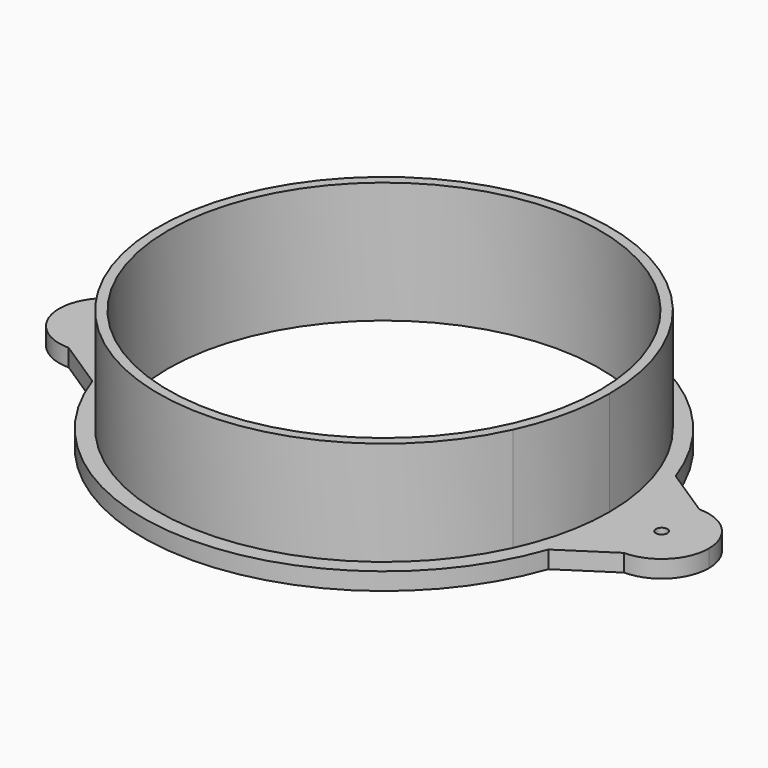
from build123d import *

# Parameters (mm, degrees)
F1_DEPTH = 5
F0_R     = 1.6686337588
F2_DEPTH = 5
F3_DEPTH = 35


with BuildPart() as f1:
    # F0 (on Top) → F1 (new body)
    with BuildSketch(Plane.XY):
        with BuildLine():
            ThreePointArc((58.9908692784, -27.2961048829), (63.4799436952, -13.9748613035), (65, 0))
            ThreePointArc((65, 0), (63.4799436952, 13.9748613035), (58.9908692784, 27.2961048829))
            ThreePointArc((58.9908692784, 27.2961048829), (35.0053794624, 54.7688178501), (0, 65))
            ThreePointArc((0, 65), (-35.0053794624, 54.7688178501), (-58.9908692784, 27.2961048829))
            ThreePointArc((-58.9908692784, 27.2961048829), (-63.4799436952, 13.9748613035), (-65, 0))
            ThreePointArc((-65, 0), (-63.4799436952, -13.9748613035), (-58.9908692784, -27.2961048829))
            ThreePointArc((-58.9908692784, -27.2961048829), (0, -65), (58.9908692784, -27.2961048829))
        make_face()
        with BuildLine():
            ThreePointArc((-62.231150434, 0), (-44.0040684729, 44.0040684729), (0, 62.231150434))
            ThreePointArc((0, 62.231150434), (44.0040684729, 44.0040684729), (62.231150434, 0))
            ThreePointArc((62.231150434, 0), (0, -62.231150434), (-62.231150434, 0))
        make_face(mode=Mode.SUBTRACT)
        with BuildLine():
            ThreePointArc((58.9908692784, 27.2961048829), (63.4799436952, 13.9748613035), (65, 0))
            Line((65, 0), (66.4206601738, 0))
            ThreePointArc((66.4206601738, 0), (67.1091179562, 4.268914411), (69.1046831796, 8.1049701726))
            ThreePointArc((69.1046831796, 8.1049701726), (67.8057771791, 15.6052670592), (65.6953330705, 22.9187912336))
            Line((65.6953330705, 22.9187912336), (58.9908692784, 27.2961048829))
        make_face()
        with BuildLine():
            Line((66.4206601738, 0), (65, 0))
            ThreePointArc((65, 0), (63.4799436952, -13.9748613035), (58.9908692784, -27.2961048829))
            Line((58.9908692784, -27.2961048829), (65.6953330705, -22.9187912336))
            ThreePointArc((65.6953330705, -22.9187912336), (67.8057771791, -15.6052670592), (69.1046831796, -8.1049701726))
            ThreePointArc((69.1046831796, -8.1049701726), (67.1091179562, -4.268914411), (66.4206601738, 0))
        make_face()
        with BuildLine():
            ThreePointArc((0, 65), (35.0053794624, 54.7688178501), (58.9908692784, 27.2961048829))
            Line((58.9908692784, 27.2961048829), (65.6953330705, 22.9187912336))
            ThreePointArc((65.6953330705, 22.9187912336), (0, 69.5783571152), (-65.6953330705, 22.9187912336))
            Line((-65.6953330705, 22.9187912336), (-58.9908692784, 27.2961048829))
            ThreePointArc((-58.9908692784, 27.2961048829), (-35.0053794624, 54.7688178501), (0, 65))
        make_face()
        with BuildLine():
            ThreePointArc((69.1046831796, 8.1049701726), (67.1091179562, 4.268914411), (66.4206601738, 0))
            ThreePointArc((66.4206601738, 0), (67.1091179562, -4.268914411), (69.1046831796, -8.1049701726))
            ThreePointArc((69.1046831796, -8.1049701726), (69.4598376886, -4.0593998478), (69.5783571152, 0))
            ThreePointArc((69.5783571152, 0), (69.4598376886, 4.0593998478), (69.1046831796, 8.1049701726))
        make_face()
        with BuildLine():
            Line((65.6953330705, -22.9187912336), (58.9908692784, -27.2961048829))
            ThreePointArc((58.9908692784, -27.2961048829), (0, -65), (-58.9908692784, -27.2961048829))
            Line((-58.9908692784, -27.2961048829), (-65.6953330705, -22.9187912336))
            ThreePointArc((-65.6953330705, -22.9187912336), (0, -69.5783571152), (65.6953330705, -22.9187912336))
        make_face()
        with BuildLine():
            Line((-65.6953330705, -22.9187912336), (-58.9908692784, -27.2961048829))
            ThreePointArc((-58.9908692784, -27.2961048829), (-63.4799436952, -13.9748613035), (-65, 0))
            Line((-65, 0), (-66.4206601738, 0))
            ThreePointArc((-66.4206601738, 0), (-67.1091179562, -4.268914411), (-69.1046831796, -8.1049701726))
            ThreePointArc((-69.1046831796, -8.1049701726), (-67.8057771791, -15.6052670592), (-65.6953330705, -22.9187912336))
        make_face()
        with BuildLine():
            ThreePointArc((-65, 0), (-63.4799436952, 13.9748613035), (-58.9908692784, 27.2961048829))
            Line((-58.9908692784, 27.2961048829), (-65.6953330705, 22.9187912336))
            ThreePointArc((-65.6953330705, 22.9187912336), (-67.8057771791, 15.6052670592), (-69.1046831796, 8.1049701726))
            ThreePointArc((-69.1046831796, 8.1049701726), (-67.1091179562, 4.268914411), (-66.4206601738, 0))
            Line((-66.4206601738, 0), (-65, 0))
        make_face()
        with BuildLine():
            ThreePointArc((-66.4206601738, 0), (-67.1091179562, 4.268914411), (-69.1046831796, 8.1049701726))
            ThreePointArc((-69.1046831796, 8.1049701726), (-69.5783571152, 0), (-69.1046831796, -8.1049701726))
            ThreePointArc((-69.1046831796, -8.1049701726), (-67.1091179562, -4.268914411), (-66.4206601738, 0))
        make_face()
    extrude(amount=F1_DEPTH)

    # F0 (on Top) → F2 (join)
    with BuildSketch(Plane.XY):
        with BuildLine():
            ThreePointArc((-69.1046831796, 8.1049701726), (-67.8057771791, 15.6052670592), (-65.6953330705, 22.9187912336))
            Line((-65.6953330705, 22.9187912336), (-80, 13.5793398262))
            ThreePointArc((-80, 13.5793398262), (-73.9033482197, 12.133808437), (-69.1046831796, 8.1049701726))
        make_face()
        with BuildLine():
            ThreePointArc((-69.1046831796, 8.1049701726), (-73.9033482197, 12.133808437), (-80, 13.5793398262))
            ThreePointArc((-80, 13.5793398262), (-89.6020432751, 9.6020432751), (-93.5793398262, 0))
            ThreePointArc((-93.5793398262, 0), (-89.6020432751, -9.6020432751), (-80, -13.5793398262))
            ThreePointArc((-80, -13.5793398262), (-73.9033482197, -12.133808437), (-69.1046831796, -8.1049701726))
            ThreePointArc((-69.1046831796, -8.1049701726), (-69.5783571152, 0), (-69.1046831796, 8.1049701726))
        make_face()
        with Locations((-80, 0)):
            Circle(F0_R, mode=Mode.SUBTRACT)
        with BuildLine():
            Line((-80, -13.5793398262), (-65.6953330705, -22.9187912336))
            ThreePointArc((-65.6953330705, -22.9187912336), (-67.8057771791, -15.6052670592), (-69.1046831796, -8.1049701726))
            ThreePointArc((-69.1046831796, -8.1049701726), (-73.9033482197, -12.133808437), (-80, -13.5793398262))
        make_face()
        with BuildLine():
            ThreePointArc((80, -13.5793398262), (73.9033482197, -12.133808437), (69.1046831796, -8.1049701726))
            ThreePointArc((69.1046831796, -8.1049701726), (67.8057771791, -15.6052670592), (65.6953330705, -22.9187912336))
            Line((65.6953330705, -22.9187912336), (80, -13.5793398262))
        make_face()
        with BuildLine():
            ThreePointArc((80, 13.5793398262), (73.9033482197, 12.133808437), (69.1046831796, 8.1049701726))
            ThreePointArc((69.1046831796, 8.1049701726), (69.4598376886, 4.0593998478), (69.5783571152, 0))
            ThreePointArc((69.5783571152, 0), (69.4598376886, -4.0593998478), (69.1046831796, -8.1049701726))
            ThreePointArc((69.1046831796, -8.1049701726), (73.9033482197, -12.133808437), (80, -13.5793398262))
            ThreePointArc((80, -13.5793398262), (89.6020432751, -9.6020432751), (93.5793398262, 0))
            ThreePointArc((93.5793398262, 0), (89.6020432751, 9.6020432751), (80, 13.5793398262))
        make_face()
        with Locations((80, 0)):
            Circle(F0_R, mode=Mode.SUBTRACT)
        with BuildLine():
            Line((80, 13.5793398262), (65.6953330705, 22.9187912336))
            ThreePointArc((65.6953330705, 22.9187912336), (67.8057771791, 15.6052670592), (69.1046831796, 8.1049701726))
            ThreePointArc((69.1046831796, 8.1049701726), (73.9033482197, 12.133808437), (80, 13.5793398262))
        make_face()
    extrude(amount=F2_DEPTH)

    # F0 (on Top) → F3 (join)
    with BuildSketch(Plane.XY):
        with BuildLine():
            ThreePointArc((58.9908692784, -27.2961048829), (63.4799436952, -13.9748613035), (65, 0))
            ThreePointArc((65, 0), (63.4799436952, 13.9748613035), (58.9908692784, 27.2961048829))
            ThreePointArc((58.9908692784, 27.2961048829), (35.0053794624, 54.7688178501), (0, 65))
            ThreePointArc((0, 65), (-35.0053794624, 54.7688178501), (-58.9908692784, 27.2961048829))
            ThreePointArc((-58.9908692784, 27.2961048829), (-63.4799436952, 13.9748613035), (-65, 0))
            ThreePointArc((-65, 0), (-63.4799436952, -13.9748613035), (-58.9908692784, -27.2961048829))
            ThreePointArc((-58.9908692784, -27.2961048829), (0, -65), (58.9908692784, -27.2961048829))
        make_face()
        with BuildLine():
            ThreePointArc((-62.231150434, 0), (-44.0040684729, 44.0040684729), (0, 62.231150434))
            ThreePointArc((0, 62.231150434), (44.0040684729, 44.0040684729), (62.231150434, 0))
            ThreePointArc((62.231150434, 0), (0, -62.231150434), (-62.231150434, 0))
        make_face(mode=Mode.SUBTRACT)
    extrude(amount=F3_DEPTH)


solid = f1.part
